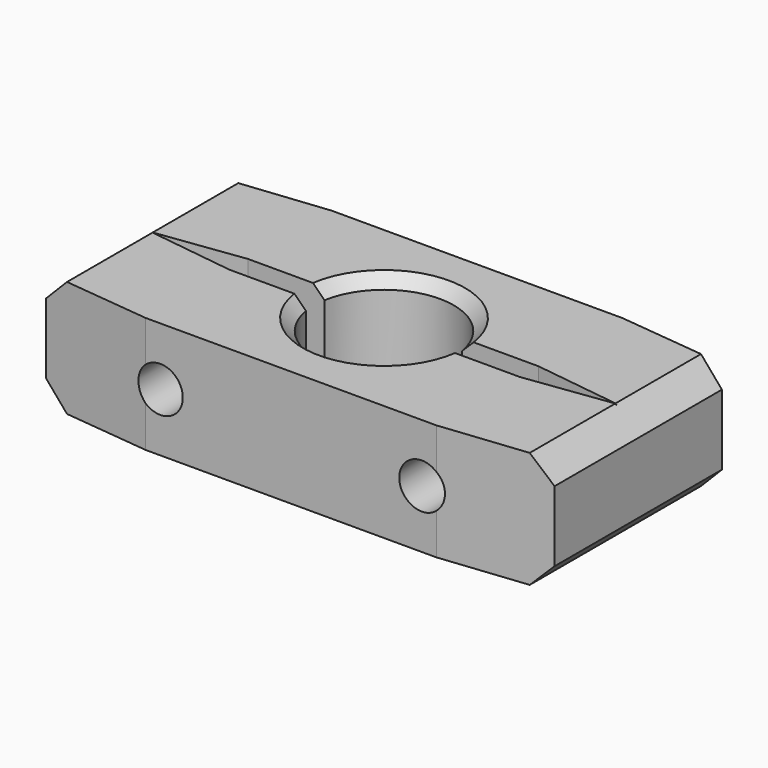
from build123d import *

# Parameters (mm, degrees)
F1_DEPTH    = 5.08
F3_D        = 3.937
F3_DEPTH    = 12.7
F3_TIP      = 1.1827941286
F4_D        = 3.937
F4_DEPTH    = 12.7
F4_START    = 1.016
F4_TIP      = 1.1827941286
F5_T1_DEPTH = 28.5747319519
F6_SIZE     = 1


# Not quite as in the source:
# - a fillet or chamfer that OpenCascade refuses, or shapes differently, is made with other operations: its cross-section is extruded or revolved along the edge and cut away or added


with BuildPart() as f1:
    # F0 (on Top) → F1 (new body, symmetric)
    with BuildSketch(Plane.XY):
        Polygon((-12.7, -10.16), (12.7, -10.16), (22.225, -9.144), (22.225, 9.144), (12.7, 10.16), (-12.7, 10.16), (-22.225, 9.144), (-22.225, -9.144), align=None)
        with BuildLine():
            ThreePointArc((6.0107370596, -1.016), (0, -6.096), (-6.0107370596, -1.016))
            Line((-6.0107370596, -1.016), (-12.7, -1.016))
            Line((-12.7, -1.016), (-20.32, 0))
            Line((-20.32, 0), (-12.7, 1.016))
            Line((-12.7, 1.016), (-6.0107370596, 1.016))
            ThreePointArc((-6.0107370596, 1.016), (0, 6.096), (6.0107370596, 1.016))
            Line((6.0107370596, 1.016), (12.7, 1.016))
            Line((12.7, 1.016), (20.32, 0))
            Line((20.32, 0), (12.7, -1.016))
            Line((12.7, -1.016), (6.0107370596, -1.016))
        make_face(mode=Mode.SUBTRACT)
    extrude(amount=F1_DEPTH, both=True)

    # F3 (one way)
    with BuildSketch(Plane.XZ):
        with Locations((-11.43, 0), (11.43, 0)):
            Circle(F3_D / 2)
    extrude(amount=-F3_DEPTH, mode=Mode.SUBTRACT)
    with Locations(Plane.XZ):
        with Locations((-11.43, 0), (11.43, 0)):
            with Locations((0, 0, -(F3_DEPTH + F3_TIP / 2))):  # 118° drill point
                Cone(0, F3_D / 2, F3_TIP, mode=Mode.SUBTRACT)

    # F4
    # its depths count from where the whole tool has entered the part; down to there all is cleared
    with Locations(Plane(origin=(0, 0, 0), x_dir=(1, 0, 0), z_dir=(0, 1, 0)).offset(-F4_START)):
        with Locations((-11.43, 0), (11.43, 0)):
            Hole(F4_D / 2, depth=F4_DEPTH)
            with Locations((0, 0, -(F4_DEPTH + F4_TIP / 2))):  # 118° drill point
                Cone(0, F4_D / 2, F4_TIP, mode=Mode.SUBTRACT)

    # F5: chamfer of 2 on 4 edges, made by hand

    # F5_s2 → F5_t1 (cut)
    with BuildSketch(Plane.XZ.offset(-14.2873659759)):
        Polygon((20.225, -5.08), (22.225, -3.08), (22.225, -5.08), align=None)
        Polygon((22.225, 3.08), (20.225, 5.08), (22.225, 5.08), align=None)
        Polygon((-22.225, 3.08), (-20.225, 5.08), (-22.225, 5.08), align=None)
        Polygon((-20.225, -5.08), (-22.225, -3.08), (-22.225, -5.08), align=None)
    extrude(amount=F5_T1_DEPTH, mode=Mode.SUBTRACT)

    # F6
    f6_edges = [f1.edges().sort_by_distance(p)[0] for p in [
        (0, -6.096, -5.08),
        (0, -6.096, 5.08),
        (0, 6.096, 5.08),
        (0, 6.096, -5.08),
    ]]
    chamfer(f6_edges, length=F6_SIZE)


solid = f1.part
